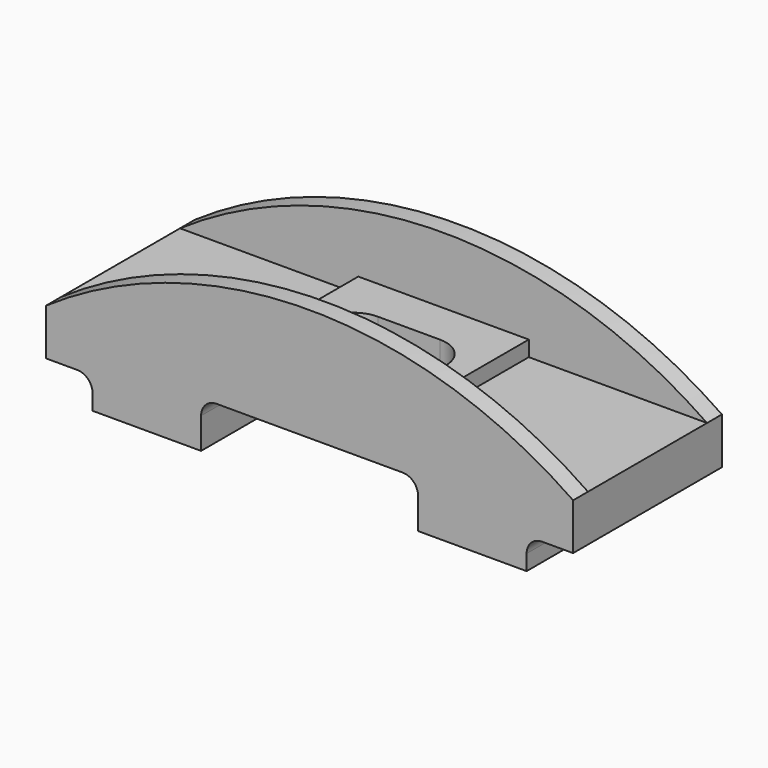
from build123d import *

# Parameters (mm, degrees)
F0_W      = 1700
F0_H      = 250
F1_DEPTH  = 600
F2_W      = 700
F2_H      = 300
F3_DEPTH  = 600.001
F4_W      = 150
F4_H      = 100
F5_DEPTH  = 600.001
F6_W      = 150
F6_H      = 100
F7_DEPTH  = 600.001
F9_DEPTH  = 60
F11_DEPTH = 60
F12_W     = 550
F12_H     = 480
F13_DEPTH = 50
F15_DEPTH = 300.001
F16_R     = 50
F17_R     = 50
F18_R     = 50
F19_R     = 50
F20_DEPTH = 300.001


# Not quite as in the source:
# - a feature names something its author has since deleted; it is built from what else it names


with BuildPart() as f1:
    # F0 (on Front) → F1 (new body)
    with BuildSketch(Plane.XZ):
        Rectangle(F0_W, F0_H)
    extrude(amount=F1_DEPTH)

    # F2 (on face) → F3 (cut, through all)
    with BuildSketch(Plane.XZ.offset(600)):
        with Locations((0, -125)):
            Rectangle(F2_W, F2_H)
    extrude(amount=-F3_DEPTH, mode=Mode.SUBTRACT)

    # F4 (on face) → F5 (cut, through all)
    with BuildSketch(Plane.XZ.offset(600)):
        with Locations((-775, -75)):
            Rectangle(F4_W, F4_H)
    extrude(amount=-F5_DEPTH, mode=Mode.SUBTRACT)

    # F6 (on face) → F7 (cut, through all)
    with BuildSketch(Plane.XZ.offset(600)):
        with Locations((775, -75)):
            Rectangle(F6_W, F6_H)
    extrude(amount=-F7_DEPTH, mode=Mode.SUBTRACT)

    # F8 (on face) → F9 (join)
    with BuildSketch(Plane.XZ.offset(600)):
        with BuildLine():
            Line((-850, 125), (850, 125))
            ThreePointArc((850, 125), (0, 389.0792905692), (-850, 125))
        make_face()
    extrude(amount=-F9_DEPTH)

    # F10 (on face) → F11 (join)
    with BuildSketch(Plane(origin=(0, 0, 0), x_dir=(-1, 0, 0), z_dir=(0, 1, 0))):
        with BuildLine():
            Line((-850, 125), (850, 125))
            ThreePointArc((850, 125), (0, 389.0792905692), (-850, 125))
        make_face()
    extrude(amount=-F11_DEPTH)

    # F12 (on face) → F13 (join)
    with BuildSketch(Plane.XY.offset(125)):
        with Locations((0, -300)):
            Rectangle(F12_W, F12_H)
    extrude(amount=F13_DEPTH)

    # F14 (on face) → F15 (cut, through all)
    with BuildSketch(Plane.XY.offset(175)):
        with BuildLine():
            ThreePointArc((-100, -200), (-200, -300), (-100, -400))
            Line((-100, -400), (100, -400))
            ThreePointArc((100, -400), (200, -300), (100, -200))
            Line((100, -200), (-100, -200))
        make_face()
    extrude(amount=-F15_DEPTH, mode=Mode.SUBTRACT)

    # F16
    f16_edges = [f1.edges().sort_by_distance(p)[0] for p in [
        (-700, -300, -25),
    ]]
    fillet(f16_edges, radius=F16_R)

    # F17
    f17_edges = [f1.edges().sort_by_distance(p)[0] for p in [
        (-350, -300, 25),
    ]]
    fillet(f17_edges, radius=F17_R)

    # F18
    f18_edges = [f1.edges().sort_by_distance(p)[0] for p in [
        (350, -300, 25),
    ]]
    fillet(f18_edges, radius=F18_R)

    # F19
    f19_edges = [f1.edges().sort_by_distance(p)[0] for p in [
        (700, -300, -25),
    ]]
    fillet(f19_edges, radius=F19_R)

    # F14 (on face) → F20 (cut, through all)
    with BuildSketch(Plane.XY.offset(175)):
        with BuildLine():
            ThreePointArc((-100, -200), (-200, -300), (-100, -400))
            Line((-100, -400), (100, -400))
            ThreePointArc((100, -400), (200, -300), (100, -200))
            Line((100, -200), (-100, -200))
        make_face()
    extrude(amount=-F20_DEPTH, mode=Mode.SUBTRACT)


solid = f1.part
